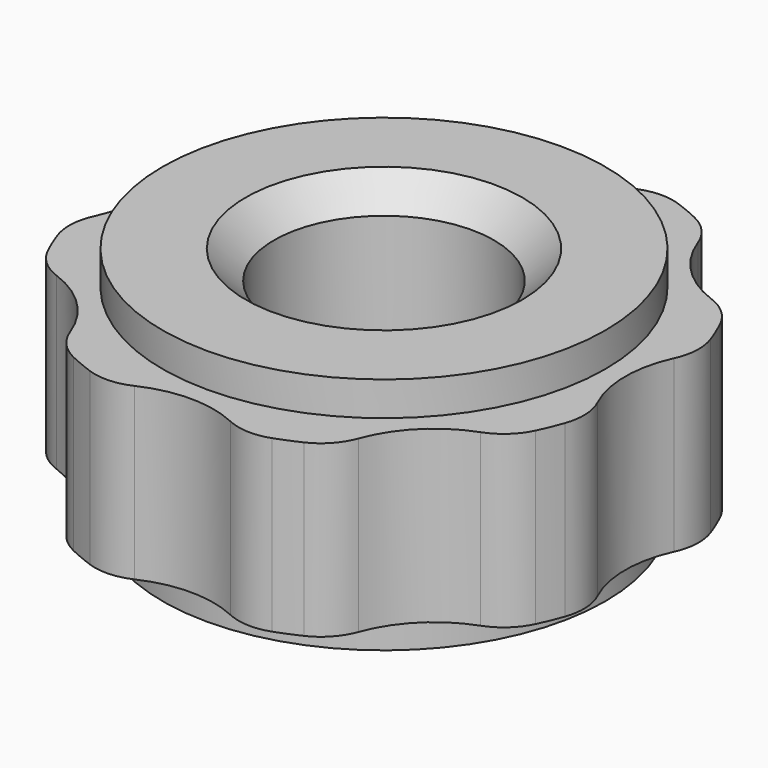
from build123d import *

# Parameters (mm, degrees)
F0_R      = 9.5
F1_DEPTH  = 6
F2_R      = 7.8
F3_DEPTH  = 1.2
F4_R      = 7.8
F5_DEPTH  = 1.2
F6_R      = 4
F7_DEPTH  = 6
F8_R      = 2
F9_R      = 3.875
F10_DEPTH = 8.401
F11_SIZE  = 1


# Not quite as in the source:
# - the program builds the solid bodies; features that only make, move or delete a surface that nothing else refers to are left out


with BuildPart() as f1:
    # F0 (on Top) → F1 (new body)
    with BuildSketch(Plane.XY):
        Circle(F0_R)
    extrude(amount=F1_DEPTH)

    # F2 (on face) → F3 (join)
    with BuildSketch(Plane.XY.offset(6)):
        Circle(F2_R)
    extrude(amount=F3_DEPTH)

    # F4 (on face) → F5 (join)
    with BuildSketch(Plane(origin=(0, 0, 0), x_dir=(1, 0, 0), z_dir=(0, 0, -1))):
        Circle(F4_R)
    extrude(amount=F5_DEPTH)

    # F6 (on face) → F7 (cut, through all)
    with BuildSketch(Plane(origin=(0, 0, 0), x_dir=(1, 0, 0), z_dir=(0, 0, -1))):
        with Locations((0, 12.5)):
            Circle(F6_R)
        with Locations((-8.8388347648, 8.8388347648)):
            Circle(F6_R)
        with Locations((-12.5, 0)):
            Circle(F6_R)
        with Locations((-8.8388347648, -8.8388347648)):
            Circle(F6_R)
        with Locations((0, -12.5)):
            Circle(F6_R)
        with Locations((8.8388347648, -8.8388347648)):
            Circle(F6_R)
        with Locations((12.5, 0)):
            Circle(F6_R)
        with Locations((8.8388347648, 8.8388347648)):
            Circle(F6_R)
    extrude(amount=-F7_DEPTH, mode=Mode.SUBTRACT)

    # F8
    f8_edges = [f1.edges().sort_by_distance(p)[0] for p in [
        (-9.22, -2.289454, 3),
        (-9.22, 2.289454, 3),
        (-4.900636, -8.138413, 3),
        (-8.138413, -4.900636, 3),
        (-8.138413, 4.900636, 3),
        (-4.900636, 8.138413, 3),
        (-2.289454, 9.22, 3),
        (2.289454, 9.22, 3),
        (8.138413, 4.900636, 3),
        (4.900636, 8.138413, 3),
        (9.22, 2.289454, 3),
        (9.22, -2.289454, 3),
        (8.138413, -4.900636, 3),
        (4.900636, -8.138413, 3),
        (2.289454, -9.22, 3),
        (-2.289454, -9.22, 3),
    ]]
    fillet(f8_edges, radius=F8_R)

    # F9 (on face) → F10 (cut, through all)
    with BuildSketch(Plane.XY.offset(7.2)):
        Circle(F9_R)
    extrude(amount=-F10_DEPTH, mode=Mode.SUBTRACT)

    # F11
    f11_edges = [f1.edges().sort_by_distance(p)[0] for p in [
        (-3.875, 0, 7.2),
        (-3.875, 0, -1.2),
    ]]
    chamfer(f11_edges, length=F11_SIZE)


solid = f1.part
